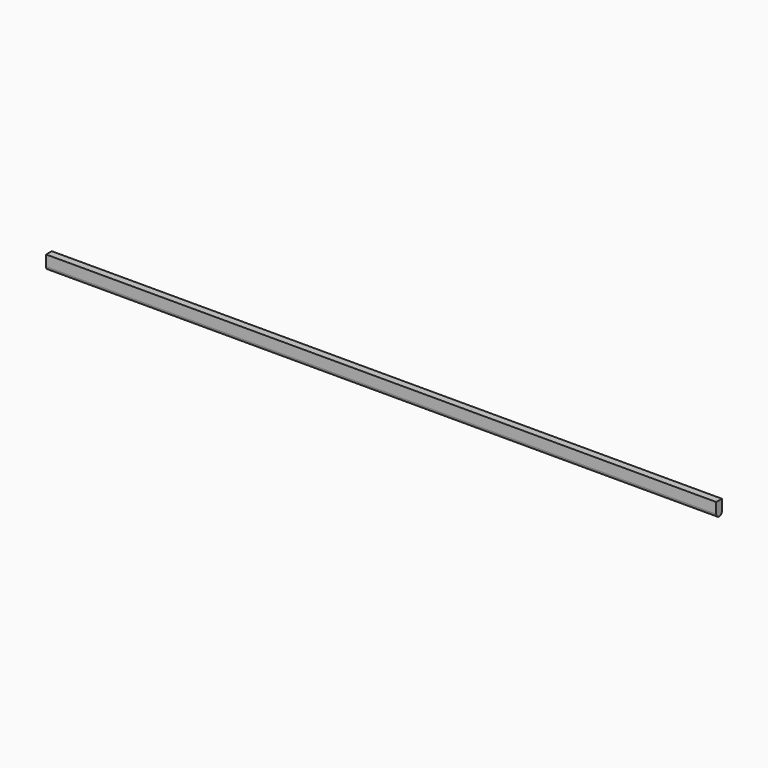
from build123d import *

# Parameters (mm, degrees)
F0_W     = 1797.05
F0_H     = 38.1
F1_DEPTH = 19.05
F2_R     = 9.52499


# Not quite as in the source:
# - a fillet or chamfer is up to 0.001 mm smaller than in the source, because OpenCascade refuses the exact size


with BuildPart() as f1:
    # F0 (on Front) → F1 (new body)
    with BuildSketch(Plane.XZ):
        with Locations((898.525, 19.05)):
            Rectangle(F0_W, F0_H)
    extrude(amount=F1_DEPTH)

    # F2 (radius 9.525 in the source; OpenCascade refuses exactly that, so slightly less here)
    f2_edges = [f1.edges().sort_by_distance(p)[0] for p in [
        (898.525, -19.05, 0),
        (898.525, 0, 0),
    ]]
    fillet(f2_edges, radius=F2_R)


solid = f1.part
